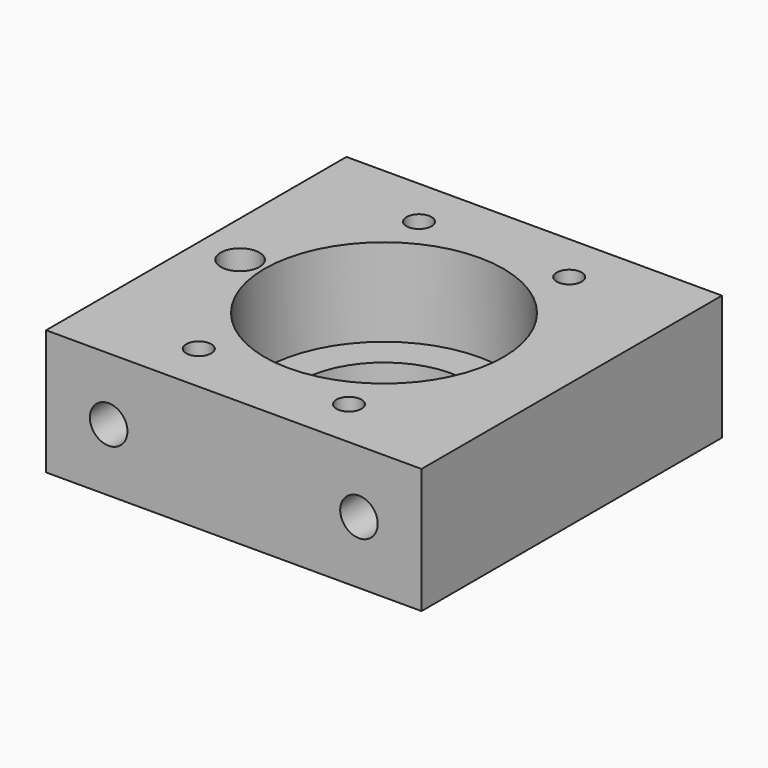
from build123d import *

# Parameters (mm, degrees)
F0_W      = 30
F0_H      = 30
F1_DEPTH  = 10
F2_R      = 9.55
F3_DEPTH  = 7
F4_R      = 6.75
F5_DEPTH  = 3
F7_DEPTH  = 10
F8_R      = 1.5
F9_DEPTH  = 8
F10_R     = 1.5
F11_DEPTH = 8
F12_R     = 1
F13_DEPTH = 10


with BuildPart() as f1:
    # F0 (on Top) → F1 (new body)
    with BuildSketch(Plane.XY):
        with Locations((15, -15)):
            Rectangle(F0_W, F0_H)
    extrude(amount=-F1_DEPTH)

    # F2 (on face) → F3 (cut)
    with BuildSketch(Plane.XY):
        with Locations((15, -15)):
            Circle(F2_R)
    extrude(amount=-F3_DEPTH, mode=Mode.SUBTRACT)

    # F4 (on face) → F5 (cut, through all)
    with BuildSketch(Plane.XY.offset(-7)):
        with Locations((15, -15)):
            Circle(F4_R)
    extrude(amount=-F5_DEPTH, mode=Mode.SUBTRACT)

    # F6 (on face) → F7 (cut, through all)
    with BuildSketch(Plane.XY):
        with BuildLine():
            ThreePointArc((1.95, -15), (3.5, -16.55), (5.05, -15))
            ThreePointArc((5.05, -15), (3.5, -13.45), (1.95, -15))
        make_face()
    extrude(amount=-F7_DEPTH, mode=Mode.SUBTRACT)

    # F8 (on face) → F9 (cut)
    with BuildSketch(Plane.XZ.offset(30)):
        with Locations((5, -5)):
            Circle(F8_R)
        with Locations((25, -5)):
            Circle(F8_R)
    extrude(amount=-F9_DEPTH, mode=Mode.SUBTRACT)

    # F10 (on face) → F11 (cut)
    with BuildSketch(Plane(origin=(0, 0, 0), x_dir=(-1, 0, 0), z_dir=(0, 1, 0))):
        with Locations((-25, -5)):
            Circle(F10_R)
        with Locations((-5, -5)):
            Circle(F10_R)
    extrude(amount=-F11_DEPTH, mode=Mode.SUBTRACT)

    # F12 (on face) → F13 (cut, through all)
    with BuildSketch(Plane(origin=(0, 0, -10), x_dir=(1, 0, 0), z_dir=(0, 0, -1))):
        with Locations((9, 4)):
            Circle(F12_R)
        with Locations((21, 4)):
            Circle(F12_R)
        with Locations((21, 26)):
            Circle(F12_R)
        with Locations((9, 26)):
            Circle(F12_R)
    extrude(amount=-F13_DEPTH, mode=Mode.SUBTRACT)


solid = f1.part
